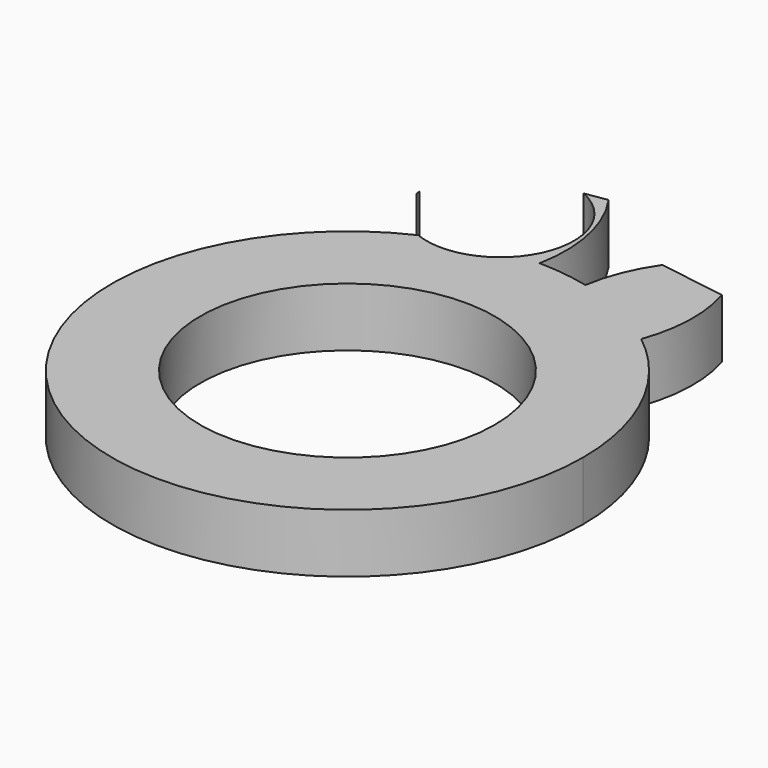
from build123d import *

# Parameters (mm, degrees)
F2_R     = 2.5
F3_DEPTH = 1


# Not quite as in the source:
# - a feature of the source that left no trace in its solid (it failed there, or was rolled back) is left out


with BuildPart() as f3:
    # F2 (on Top) → F3 (new body)
    with BuildSketch(Plane.XY):
        with BuildLine():
            ThreePointArc((-1.6960043415, 3.6226467222), (-2.1466232359, -3.3752049839), (4, 0))
            ThreePointArc((4, 0), (3.7786523245, 1.3121686669), (3.1391066948, 2.4791145917))
            ThreePointArc((3.1391066948, 2.4791145917), (2.8274967449, 2.8293571986), (2.4770492462, 3.1407367021))
            ThreePointArc((2.4770492462, 3.1407367021), (1.7443008848, 3.5996408742), (0.9300595273, 3.8903713545))
            ThreePointArc((0.9300595273, 3.8903713545), (0.5005649816, 3.9685557447), (0.0651081325, 3.9994700813))
            ThreePointArc((0.0651081325, 3.9994700813), (-0.0993482735, 3.9987660497), (-0.2636367411, 3.9913025028))
            ThreePointArc((-0.2636367411, 3.9913025028), (-0.9194446737, 3.572391456), (-1.6960043415, 3.6226467222))
        make_face()
        Circle(F2_R, mode=Mode.SUBTRACT)
        with BuildLine():
            ThreePointArc((0.9300595273, 3.8903713545), (1.7443008848, 3.5996408742), (2.4770492462, 3.1407367021))
            ThreePointArc((2.4770492462, 3.1407367021), (2.6347989126, 3.9640717606), (2.5237715391, 4.7949980498))
            Line((2.5237715391, 4.7949980498), (1.3669232641, 4.9782248164))
            ThreePointArc((1.3669232641, 4.9782248164), (1.0867126989, 4.4591073757), (0.9300595273, 3.8903713545))
        make_face()
        with BuildLine():
            ThreePointArc((-0.733402564, 5.9296250647), (-0.0161783263, 5.0773625262), (-0.2636367411, 3.9913025028))
            ThreePointArc((-0.2636367411, 3.9913025028), (-0.0993482735, 3.9987660497), (0.0651081325, 3.9994700813))
            ThreePointArc((0.0651081325, 3.9994700813), (0.0562243119, 5.0370730396), (-0.3557009583, 5.9894471221))
            Line((-0.3557009583, 5.9894471221), (-0.733402564, 5.9296250647))
        make_face()
    extrude(amount=F3_DEPTH)


with BuildPart() as f3b:
    # F2 (on Top) → F3, piece 2 (new body)
    with BuildSketch(Plane.XY):
        with BuildLine():
            ThreePointArc((-2.4696169155, 4.6145588285), (-2.4642610911, 4.5790010988), (-2.4578846973, 4.5436121372))
            ThreePointArc((-2.4578846973, 4.5436121372), (-2.4635067961, 4.579125834), (-2.4696169155, 4.6145588285))
        make_face()
    extrude(amount=F3_DEPTH)


solid = Compound([f3.part, f3b.part])
